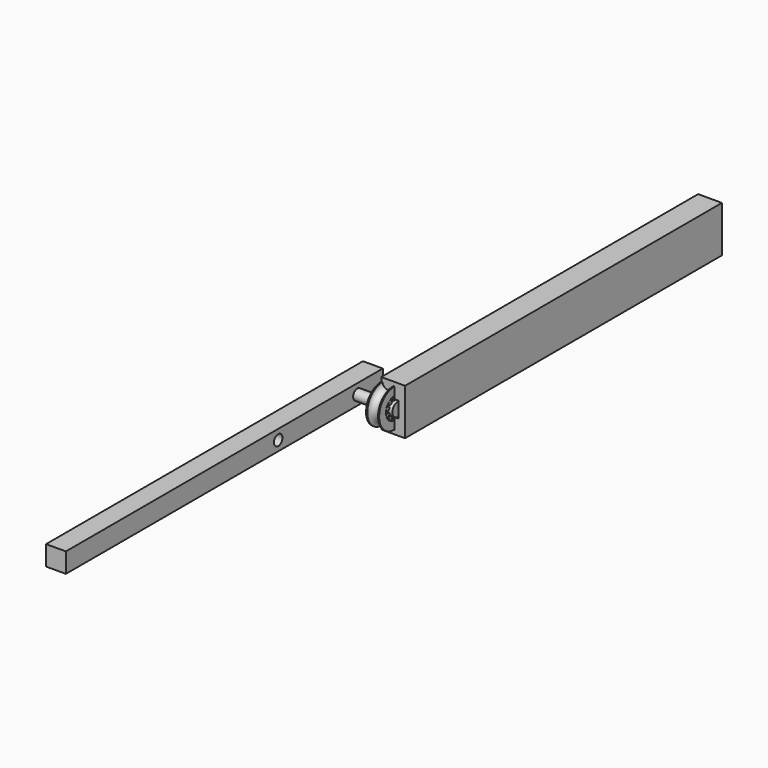
from build123d import *

# Parameters (mm, degrees)
F1_DEPTH = 300
F4_R     = 4.025
F5_DEPTH = 18.001
F6_W     = 2.4
F6_H     = 5
F8_W     = 300
F8_H     = 15
F8_R     = 4.025
F9_DEPTH = 15


with BuildPart() as f1:
    # F0 (on Front) → F1 (new body)
    with BuildSketch(Plane.XZ):
        Polygon((5, 35), (0, 35), (-13, 35), (-13, 32), (-12, 32), (-4, 32), (-3, 32), (-3, 23.5), (0, 23.5), (0, 17.5), (0, 11.5), (-3, 11.5), (-3, 3), (-4, 3), (-12, 3), (-13, 3), (-13, 0), (0, 0), (5, 0), align=None)
        with BuildLine():
            Line((-4, 32), (-12, 32))
            ThreePointArc((-12, 32), (-8, 28), (-4, 32))
        make_face()
        with BuildLine():
            ThreePointArc((-4, 3), (-8, 7), (-12, 3))
            Line((-12, 3), (-4, 3))
        make_face()
    extrude(amount=-F1_DEPTH)


with BuildPart() as f3:
    # F2 (on Front) → F3 (revolve)
    with BuildSketch(Plane.XZ):
        with BuildLine():
            ThreePointArc((-3.9012196936, 31.9), (-8, 27.9), (-12.0987803064, 31.9))
            Line((-12.0987803064, 31.9), (-13, 31.9))
            Line((-13, 31.9), (-13, 17.5))
            Line((-13, 17.5), (-3.1, 17.5))
            Line((-3.1, 17.5), (-3.1, 31.9))
            Line((-3.1, 31.9), (-3.9012196936, 31.9))
        make_face()
    revolve(axis=Axis((-8.05, 0, 17.5), (1, 0, 0)))

    # F4 (on face) → F5 (cut, through all)
    with BuildSketch(Plane(origin=(-13, 0, 0), x_dir=(0, -1, 0), z_dir=(-1, 0, 0))):
        with BuildLine():
            ThreePointArc((2.9389262209, 21.5450850013), (2.607078685, 23.6402883924), (4.7022820788, 23.9721359111))
            ThreePointArc((4.7022820788, 23.9721359111), (2.4721359905, 25.1084521188), (0, 25.5))
            ThreePointArc((0, 25.5), (1.0606601718, 25.0606601718), (1.5, 24))
            ThreePointArc((1.5, 24), (1.0606601843, 22.9393398407), (3.53e-08, 22.5))
            ThreePointArc((3.53e-08, 22.5), (1.5450849648, 22.2552825838), (2.9389262209, 21.5450850013))
        make_face()
        with BuildLine():
            ThreePointArc((4.7552826033, 19.0450849048), (5.7183418168, 20.9351952224), (7.6084521213, 19.972135983))
            ThreePointArc((7.6084521213, 19.972135983), (6.4721359683, 22.202282), (4.7022820788, 23.9721359111))
            ThreePointArc((4.7022820788, 23.9721359111), (5.1571139431, 23.4395961798), (5.3206041399, 22.7586104634))
            ThreePointArc((5.3206041399, 22.7586104634), (4.5015898672, 21.4221006658), (2.9389262209, 21.5450850013))
            ThreePointArc((2.9389262209, 21.5450850013), (4.0450849779, 20.4389262532), (4.7552826033, 19.0450849048))
        make_face()
        with BuildLine():
            ThreePointArc((7.6084521213, 15.027864017), (7.9015067225, 16.2485242651), (8, 17.5))
            ThreePointArc((8, 17.5), (7.9015067225, 18.7514757349), (7.6084521213, 19.972135983))
            ThreePointArc((7.6084521213, 19.972135983), (7.6633998645, 19.7432621756), (7.6818673559, 19.5086104634))
            ThreePointArc((7.6818673559, 19.5086104634), (6.4165190883, 18.0270779581), (4.7552826033, 19.0450849048))
            ThreePointArc((4.7552826033, 19.0450849048), (4.9384417085, 18.2821722904), (5, 17.5))
            ThreePointArc((5, 17.5), (4.9384416988, 16.7178276482), (4.7552825648, 15.9549149769))
            ThreePointArc((4.7552825648, 15.9549149769), (6.4165190269, 16.9729220517), (7.6818673559, 15.4913895366))
            ThreePointArc((7.6818673559, 15.4913895366), (7.6633998645, 15.2567378244), (7.6084521213, 15.027864017))
        make_face()
        with BuildLine():
            ThreePointArc((3.53e-08, 22.5), (-1.5, 23.9999999824), (0, 25.5))
            ThreePointArc((0, 25.5), (-2.4721359511, 25.1084521316), (-4.7022820116, 23.9721359599))
            ThreePointArc((-4.7022820116, 23.9721359599), (-3.1396183866, 24.0951202478), (-2.3206041399, 22.7586104634))
            ThreePointArc((-2.3206041399, 22.7586104634), (-2.4840943313, 22.0776247576), (-2.938926182, 21.5450850296))
            ThreePointArc((-2.938926182, 21.5450850296), (-1.5450849084, 22.2552826021), (3.53e-08, 22.5))
        make_face()
        with BuildLine():
            ThreePointArc((-2.938926182, 21.5450850296), (-5.034129605, 21.8769325486), (-4.7022820116, 23.9721359599))
            ThreePointArc((-4.7022820116, 23.9721359599), (-6.4721359439, 22.2022820336), (-7.6084521213, 19.972135983))
            ThreePointArc((-7.6084521213, 19.972135983), (-5.9472156438, 20.990142972), (-4.6818673559, 19.5086104634))
            ThreePointArc((-4.6818673559, 19.5086104634), (-4.7003348505, 19.273958731), (-4.7552826033, 19.0450849048))
            ThreePointArc((-4.7552826033, 19.0450849048), (-4.0450849637, 20.4389262727), (-2.938926182, 21.5450850296))
        make_face()
        with BuildLine():
            ThreePointArc((-4.7552826033, 19.0450849048), (-6.645392895, 18.0820257044), (-7.6084521213, 19.972135983))
            ThreePointArc((-7.6084521213, 19.972135983), (-8, 17.5000000186), (-7.6084521328, 15.0278640524))
            ThreePointArc((-7.6084521328, 15.0278640524), (-6.6453928634, 16.9179743058), (-4.7552825942, 15.9549150673))
            ThreePointArc((-4.7552825942, 15.9549150673), (-5, 17.4999999853), (-4.7552826033, 19.0450849048))
        make_face()
        with BuildLine():
            ThreePointArc((-7.6084521328, 15.0278640524), (-6.4721359523, 12.797717978), (-4.7022820047, 11.0278640351))
            ThreePointArc((-4.7022820047, 11.0278640351), (-5.0341296075, 13.1230674479), (-2.938926182, 13.4549149704))
            ThreePointArc((-2.938926182, 13.4549149704), (-4.0450849551, 14.5610737155), (-4.7552825942, 15.9549150673))
            ThreePointArc((-4.7552825942, 15.9549150673), (-4.7003348482, 15.7260412545), (-4.6818673559, 15.4913895366))
            ThreePointArc((-4.6818673559, 15.4913895366), (-5.9472156622, 14.0098570251), (-7.6084521328, 15.0278640524))
        make_face()
        with BuildLine():
            ThreePointArc((-4.7022820047, 11.0278640351), (-2.4721359497, 9.8915478679), (-5.8e-09, 9.5))
            ThreePointArc((-5.8e-09, 9.5), (-1.5, 11.0000000029), (0, 12.5))
            ThreePointArc((0, 12.5), (-1.5450849252, 12.7447174033), (-2.938926182, 13.4549149704))
            ThreePointArc((-2.938926182, 13.4549149704), (-2.4840943313, 12.9223752424), (-2.3206041399, 12.2413895366))
            ThreePointArc((-2.3206041399, 12.2413895366), (-3.1396183828, 10.9048797541), (-4.7022820047, 11.0278640351))
        make_face()
        with BuildLine():
            ThreePointArc((-5.8e-09, 9.5), (2.4721359416, 9.8915478653), (4.7022820002, 11.0278640318))
            ThreePointArc((4.7022820002, 11.0278640318), (2.6070786407, 11.3597116687), (2.9389262644, 13.4549150303))
            ThreePointArc((2.9389262644, 13.4549150303), (1.5450849736, 12.7447174191), (0, 12.5))
            ThreePointArc((0, 12.5), (1.0606601718, 12.0606601718), (1.5, 11))
            ThreePointArc((1.5, 11), (1.0606601697, 9.9393398262), (-5.8e-09, 9.5))
        make_face()
        with BuildLine():
            ThreePointArc((4.7022820002, 11.0278640318), (6.4721359397, 12.7977179606), (7.6084521213, 15.027864017))
            ThreePointArc((7.6084521213, 15.027864017), (5.7183418759, 14.0648047584), (4.7552825648, 15.9549149769))
            ThreePointArc((4.7552825648, 15.9549149769), (4.0450849571, 14.5610737183), (2.9389262644, 13.4549150303))
            ThreePointArc((2.9389262644, 13.4549150303), (4.5015898911, 13.577899322), (5.3206041399, 12.2413895366))
            ThreePointArc((5.3206041399, 12.2413895366), (5.1571139211, 11.5604037769), (4.7022820002, 11.0278640318))
        make_face()
        with Locations((0, 17.5)):
            Circle(F4_R)
    extrude(amount=-F5_DEPTH, mode=Mode.SUBTRACT)


with BuildPart() as f7:
    # F6 (on Front) → F7 (revolve)
    with BuildSketch(Plane.XZ):
        Polygon((-3.1, 17.5), (-3, 17.5), (-3, 22.5), (-3.1, 22.5), (-3.1, 21.5), (-13, 21.5), (-31.0829728842, 21.5), (-31.0829728842, 17.5), (-13, 17.5), align=None)
        with Locations((-1.8, 20)):
            Rectangle(F6_W, F6_H)
    revolve(axis=Axis((-17.0914864421, 0, 17.5), (1, 0, 0)))


with BuildPart() as f9:
    # F8 (on face) → F9 (new body)
    with BuildSketch(Plane(origin=(-31.0829728842, 0, 0), x_dir=(0, -1, 0), z_dir=(-1, 0, 0))):
        with Locations((125.975, 17.525)):
            Rectangle(F8_W, F8_H)
        with Locations((0, 17.5)):
            Circle(F8_R, mode=Mode.SUBTRACT)
        with Locations((75, 17.5)):
            Circle(F8_R, mode=Mode.SUBTRACT)
    extrude(amount=F9_DEPTH)


solid = Compound([f1.part, f3.part, f7.part, f9.part])
